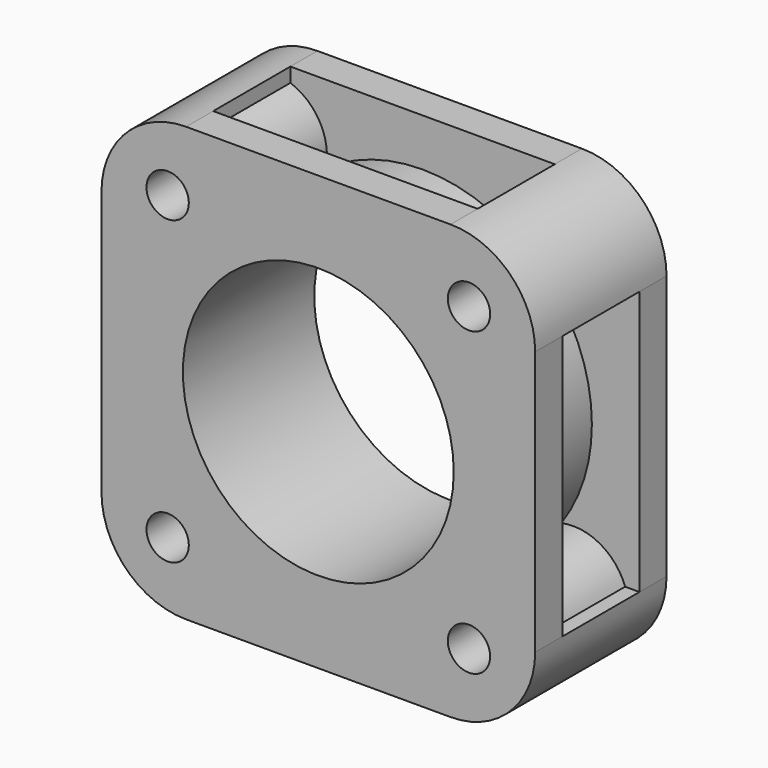
from build123d import *

# Parameters (mm, degrees)
F0_R     = 1.5875
F0_R_2   = 10.16
F1_DEPTH = 12.319
F2_T     = 2.54


# Not quite as in the source:
# - a shell that OpenCascade refuses in one call is made with other operations: the cavity is built on its own and cut out


with BuildPart() as f1:
    # F0 (on Front) → F1 (new body)
    with BuildSketch(Plane.XZ):
        with BuildLine():
            Line((9.9187, 16.2687), (-9.9187, 16.2687))
            ThreePointArc((-9.9187, 16.2687), (-14.4088280605, 14.4088280605), (-16.2687, 9.9187))
            Line((-16.2687, 9.9187), (-16.2687, -9.9187))
            ThreePointArc((-16.2687, -9.9187), (-14.4088280605, -14.4088280605), (-9.9187, -16.2687))
            Line((-9.9187, -16.2687), (9.9187, -16.2687))
            ThreePointArc((9.9187, -16.2687), (14.4088280605, -14.4088280605), (16.2687, -9.9187))
            Line((16.2687, -9.9187), (16.2687, 9.9187))
            ThreePointArc((16.2687, 9.9187), (14.4088280605, 14.4088280605), (9.9187, 16.2687))
        make_face()
        with Locations((-11.303, -11.303)):
            Circle(F0_R, mode=Mode.SUBTRACT)
        with Locations((11.303, -11.303)):
            Circle(F0_R, mode=Mode.SUBTRACT)
        Circle(F0_R_2, mode=Mode.SUBTRACT)
        with Locations((-11.303, 11.303)):
            Circle(F0_R, mode=Mode.SUBTRACT)
        with Locations((11.303, 11.303)):
            Circle(F0_R, mode=Mode.SUBTRACT)
    extrude(amount=F1_DEPTH)

    # F2: shell of thickness 2.54, made by hand


with BuildPart() as f2_core1:
    # F2_t2: copy of F1
    add(f1.part)

    # the walls: a layer under each face that stays
    f2_faces = [f2_core1.faces().sort_by_distance(p)[0] for p in [
        (14.4088280605, -6.1595, 14.4088280605),
        (-14.4088280605, -6.1595, 14.4088280605),
        (-14.4088280605, -6.1595, -14.4088280605),
        (14.4088280605, -6.1595, -14.4088280605),
        (-12.8905, -6.1595, -11.303),
        (9.7155, -6.1595, -11.303),
        (-10.16, -6.1595, 0),
        (-12.8905, -6.1595, 11.303),
        (9.7155, -6.1595, 11.303),
        (-10.8458, 0, 0),
        (-10.8458, -12.319, 0),
    ]]
    thicken(f2_faces, amount=-F2_T, mode=Mode.SUBTRACT)


with BuildPart() as f1_1:
    add(f1.part)

    # what is left inside the walls is the cavity
    f2_cavity = [f2_core1.part.solids().sort_by_distance(p)[0] for p in [
        (16.2433, -7.366, 0),
        (0, -7.366, 16.2433),
        (0, -7.366, -16.2433),
        (-16.2433, -7.366, 0),
    ]]
    add(f2_cavity, mode=Mode.SUBTRACT)


solid = f1_1.part
